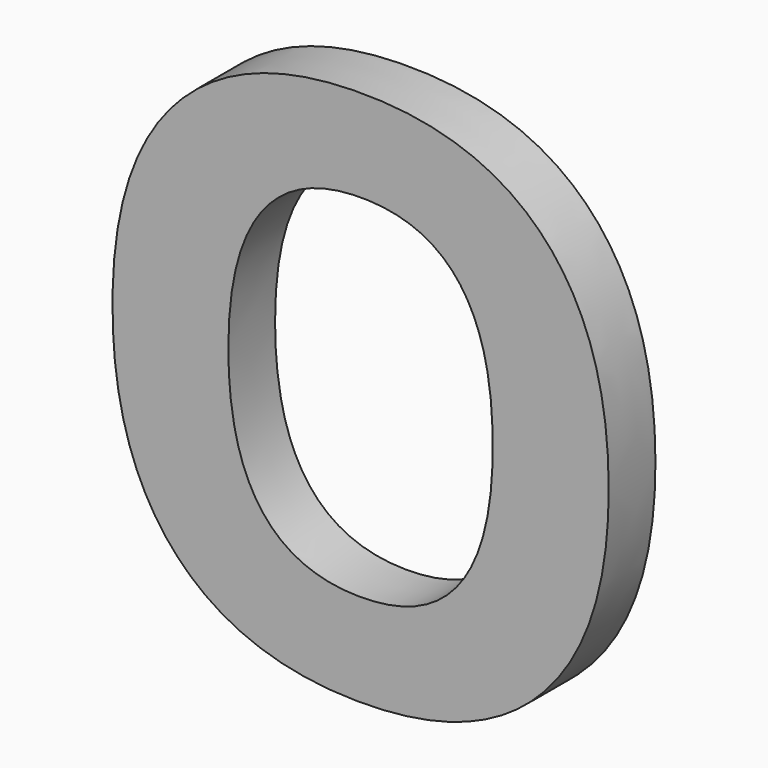
from build123d import *

# Parameters (mm, degrees)
F0_TEXT_SIZE = 62.5
F1_DEPTH     = 5


# Not quite as in the source:
# - Text() gives the source's letters only with a copy of the font that has no kerning and outlines rounded to 1/6400 em; it was checked with that copy


with BuildPart() as f1:
    # F0 (on Front) → F1 (new body)
    with BuildSketch(Plane.XZ):
        with Locations((-61.5081520345, 8.0706522811)):
            Text('O', F0_TEXT_SIZE, font='Open Sans', font_style=FontStyle.BOLD, text_align=(TextAlign.LEFT, TextAlign.BOTTOM))
    extrude(amount=F1_DEPTH)


solid = f1.part
